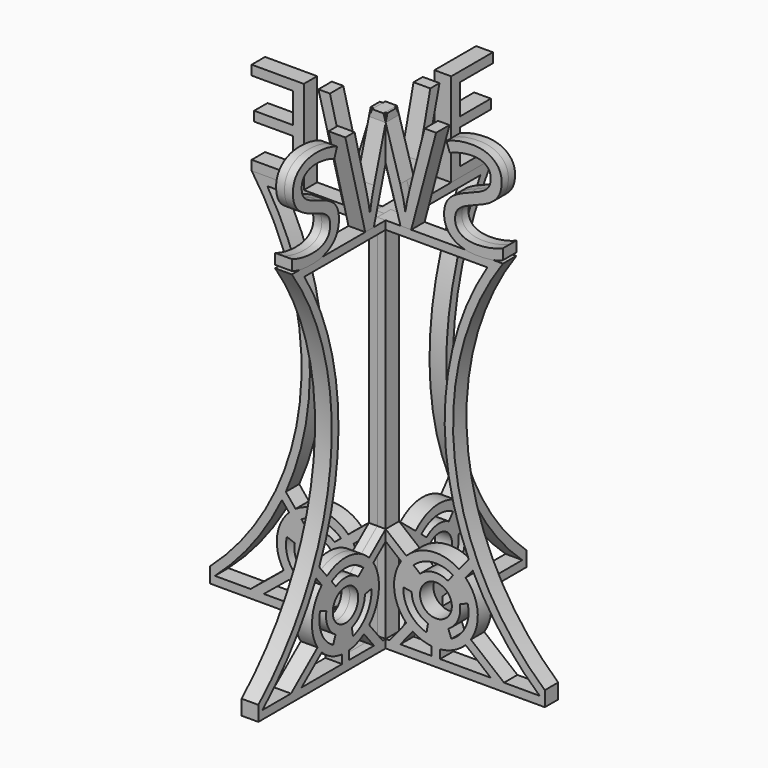
from build123d import *

# Parameters (mm, degrees)
F0_R          = 3.8
F1_DEPTH      = 2
F1_DEPTH_BACK = 2
F3_COUNT      = 4
F3_ANGLE      = 270
F4_TEXT_SIZE  = 31.2607239268
F5_DEPTH      = 2
F5_DEPTH_BACK = 2
F7_COUNT      = 2
F7_ANGLE      = 90


# Not quite as in the source:
# - Text() gives the source's letters only with a copy of the font that has no kerning and outlines rounded to 1/6400 em; it was checked with that copy


with BuildPart() as f1:
    # F0 (on Right) → F1 (new body, two sides)
    with BuildSketch(Plane.YZ) as f1_sk:
        with BuildLine():
            Line((0, 90), (-30, 90))
            ThreePointArc((-30, 90), (-18.520884582, 44.8859257291), (-40, 3.5858362744))
            Line((-40, 3.5858362744), (-40, 0))
            Line((-40, 0), (0, 0))
            Line((0, 0), (0, 90))
        make_face()
        with BuildLine():
            Line((-15, 2), (-27.1014528213, 2))
            Line((-27.1014528213, 2), (-21.0710678119, 6.9289321881))
            ThreePointArc((-21.0710678119, 6.9289321881), (-18.2845554854, 4.9643713947), (-15, 4.0501256289))
            Line((-15, 4.0501256289), (-15, 2))
        make_face(mode=Mode.SUBTRACT)
        with BuildLine():
            Line((-30.2617509523, 2), (-38.7738357231, 2))
            ThreePointArc((-38.7738357231, 2), (-29.7206024764, 11.7797762364), (-22.7714391277, 23.1514157051))
            Line((-22.7714391277, 23.1514157051), (-21.0710678119, 21.0710678119))
            ThreePointArc((-21.0710678119, 21.0710678119), (-23.9498743711, 15), (-22.3367711836, 8.4774782723))
            Line((-22.3367711836, 8.4774782723), (-30.2617509523, 2))
        make_face(mode=Mode.SUBTRACT)
        with BuildLine():
            ThreePointArc((-17.6744998657, 7.1197346899), (-21.1111382964, 10.7950488102), (-21.5884938721, 15.80409555))
            Line((-21.5884938721, 15.80409555), (-19.697057702, 15.0879032767))
            ThreePointArc((-19.697057702, 15.0879032767), (-19.2877695025, 11.6168311666), (-16.9583075924, 9.0111708599))
            Line((-16.9583075924, 9.0111708599), (-17.6744998657, 7.1197346899))
        make_face(mode=Mode.SUBTRACT)
        with Locations((-14, 14)):
            Circle(F0_R, mode=Mode.SUBTRACT)
        with BuildLine():
            ThreePointArc((-18.1212346105, 20.6223428849), (-13.22, 21.7609020094), (-8.6433604868, 19.6697806947))
            Line((-8.6433604868, 19.6697806947), (-10.2093192745, 18.3898450584))
            ThreePointArc((-10.2093192745, 18.3898450584), (-13.42, 19.7709271352), (-16.8412989742, 19.0563840973))
            Line((-16.8412989742, 19.0563840973), (-18.1212346105, 20.6223428849))
        make_face(mode=Mode.SUBTRACT)
        with BuildLine():
            Line((-8.4774782723, 5.6632288164), (-5.4833400212, 2))
            Line((-5.4833400212, 2), (-13, 2))
            Line((-13, 2), (-13, 4.0501256289))
            ThreePointArc((-13, 4.0501256289), (-10.640483979, 4.5812075028), (-8.4774782723, 5.6632288164))
        make_face(mode=Mode.SUBTRACT)
        with BuildLine():
            ThreePointArc((-6.2042655239, 14.2579224252), (-7.6688617036, 9.4440491803), (-11.7681456411, 6.5261237553))
            Line((-11.7681456411, 6.5261237553), (-12.0936230235, 8.5222516648))
            ThreePointArc((-12.0936230235, 8.5222516648), (-9.2922304975, 10.6122416982), (-8.2003934334, 13.9324450428))
            Line((-8.2003934334, 13.9324450428), (-6.2042655239, 14.2579224252))
        make_face(mode=Mode.SUBTRACT)
        with BuildLine():
            Line((-2.9002719157, 2), (-6.9289321881, 6.9289321881))
            ThreePointArc((-6.9289321881, 6.9289321881), (-4.0501256289, 13), (-5.6632288164, 19.5225217277))
            Line((-5.6632288164, 19.5225217277), (-2, 22.5166599788))
            Line((-2, 22.5166599788), (-2, 2))
            Line((-2, 2), (-2.9002719157, 2))
        make_face(mode=Mode.SUBTRACT)
        with BuildLine():
            Line((-26.2754019968, 88), (-2, 88))
            Line((-2, 88), (-2, 25.0997280843))
            Line((-2, 25.0997280843), (-6.9289321881, 21.0710678119))
            ThreePointArc((-6.9289321881, 21.0710678119), (-13, 23.9498743711), (-19.5225217277, 22.3367711836))
            Line((-19.5225217277, 22.3367711836), (-21.8385142186, 25.1703111606))
            ThreePointArc((-21.8385142186, 25.1703111606), (-16.2551126211, 57.1361039222), (-26.2754019968, 88))
        make_face(mode=Mode.SUBTRACT)
    extrude(amount=F1_DEPTH)
    extrude(f1_sk.sketch, amount=-F1_DEPTH_BACK)


with BuildPart() as f3_1:
    # F3: instance of F1
    add(f1.part.rotate(Axis((0, 0, 26.2590656057), (0, 0, -1)), 1 * F3_ANGLE / (F3_COUNT - 1)))


with BuildPart() as f3_2:
    # F3: instance of F1
    add(f1.part.rotate(Axis((0, 0, 26.2590656057), (0, 0, -1)), 2 * F3_ANGLE / (F3_COUNT - 1)))


with BuildPart() as f3_3:
    # F3: instance of F1
    add(f1.part.rotate(Axis((0, 0, 26.2590656057), (0, 0, -1)), 3 * F3_ANGLE / (F3_COUNT - 1)))


with BuildPart() as f5:
    # F4 (on Right) → F5 (new body, two sides)
    with BuildSketch(Plane.YZ) as f5_sk:
        with Locations((-31.6080485763, 90)):
            Text('SWE', F4_TEXT_SIZE, font='Open Sans', text_align=(TextAlign.LEFT, TextAlign.BOTTOM))
    extrude(amount=F5_DEPTH)
    extrude(f5_sk.sketch, amount=-F5_DEPTH_BACK)


with BuildPart() as f7_1:
    # F7: instance of F5
    add(f5.part.rotate(Axis((0, 0, 82.2183042765), (0, 0, 1)), 1 * F7_ANGLE / (F7_COUNT - 1)))


solid = Compound([f1.part, f3_1.part, f3_2.part, f3_3.part, f5.part, f7_1.part])
